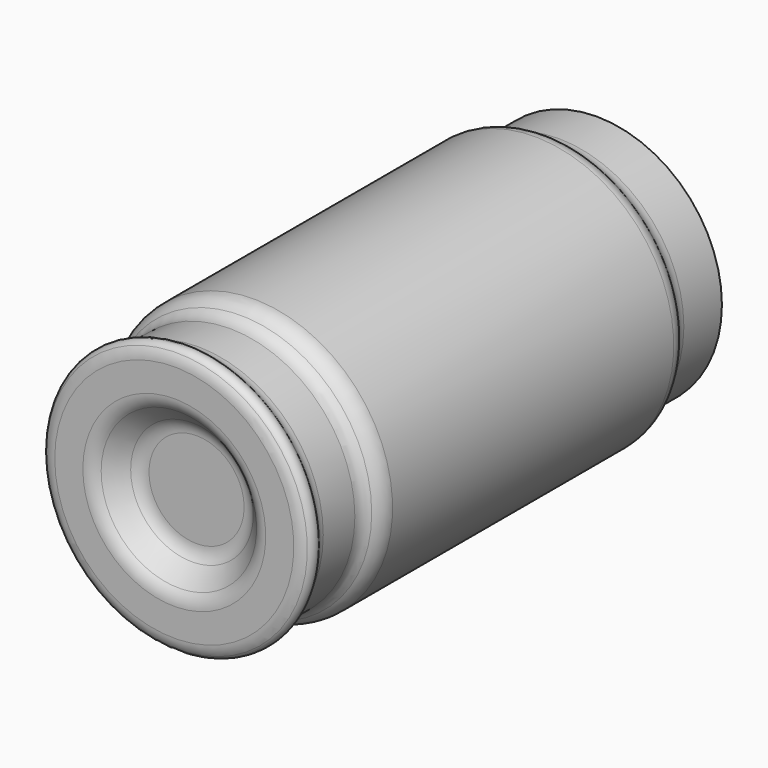
from build123d import *


# Not quite as in the source:
# - ends of sketch curves that miss each other by under 0.0002 mm in the source are joined


with BuildPart() as f1:
    # F0 (on Top) → F1 (revolve)
    with BuildSketch(Plane.XY):
        with BuildLine():
            Line((-50, 0), (-49.25, 0))
            Line((-49.25, 0), (-49.25, 67.100505))
            ThreePointArc((-49.25, 67.100505), (-48.7742470782, 69.4922764523), (-47.4194173824, 71.5199223824))
            Line((-47.4194173824, 71.5199223824), (-46.519922, 72.419417))
            ThreePointArc((-46.519922, 72.419417), (-44.839933623, 74.9336983992), (-44.25, 77.899495))
            Line((-44.25, 77.899495), (-44.25, 95))
            Line((-44.25, 95), (-45, 95))
            Line((-45, 95), (-45, 77.899495))
            ThreePointArc((-45, 77.899495), (-45.5328434077, 75.2207106468), (-47.0502530317, 72.9497470317))
            Line((-47.0502530317, 72.9497470317), (-47.949748, 72.050252))
            ThreePointArc((-47.949748, 72.050252), (-49.4671568629, 69.7792886999), (-50, 67.100505))
            Line((-50, 67.100505), (-50, 0))
        make_face()
        with BuildLine():
            Line((0, -85), (0, -84.25))
            Line((0, -84.25), (-17.100505, -84.25))
            ThreePointArc((-17.100505, -84.25), (-20.0663019275, -84.8399337583), (-22.5805830542, -86.5199229458))
            Line((-22.5805830542, -86.5199229458), (-28.480078, -92.419418))
            ThreePointArc((-28.480078, -92.419418), (-30.5077238744, -93.7742472135), (-32.899495, -94.25))
            Line((-32.899495, -94.25), (-43, -94.25))
            ThreePointArc((-43, -94.25), (-44.8261945083, -93.97724967), (-46.4929985671, -93.1828043577))
            ThreePointArc((-46.4929985671, -93.1828043577), (-47.4751196599, -91.5330711078), (-46.8265097577, -89.7260052423))
            Line((-46.8265097577, -89.7260052423), (-46.300253, -89.199748))
            ThreePointArc((-46.300253, -89.199748), (-44.7828434077, -86.9287843532), (-44.25, -84.25))
            Line((-44.25, -84.25), (-44.25, -70.04899))
            ThreePointArc((-44.25, -70.04899), (-44.9057111418, -67.090950297), (-46.7499996812, -64.6870876202))
            ThreePointArc((-46.7499996812, -64.6870876202), (-48.5942887223, -62.2832249943), (-49.25, -59.325185))
            Line((-49.25, -59.325185), (-49.25, 0))
            Line((-49.25, 0), (-50, 0))
            Line((-50, 0), (-50, -59.325185))
            ThreePointArc((-50, -59.325185), (-49.2740340482, -62.6001576243), (-47.2321430477, -65.2615770568))
            ThreePointArc((-47.2321430477, -65.2615770568), (-45.5854564677, -67.4078829271), (-45, -70.04899))
            Line((-45, -70.04899), (-45, -84.25))
            ThreePointArc((-45, -84.25), (-45.4757530571, -86.6417717789), (-46.8305831176, -88.6694178824))
            Line((-46.8305831176, -88.6694178824), (-47.35684, -89.195675))
            ThreePointArc((-47.35684, -89.195675), (-48.2216532424, -91.6050961743), (-46.9121588277, -93.8047407443))
            ThreePointArc((-46.9121588277, -93.8047407443), (-45.0453380572, -94.6945195669), (-43, -95))
            Line((-43, -95), (-32.899495, -95))
            ThreePointArc((-32.899495, -95), (-30.2207113001, -94.4671568629), (-27.9497480317, -92.9497479683))
            Line((-27.9497480317, -92.9497479683), (-22.050253, -87.050253))
            ThreePointArc((-22.050253, -87.050253), (-19.7792893532, -85.5328434077), (-17.100505, -85))
            Line((-17.100505, -85), (0, -85))
        make_face()
    revolve(axis=Axis((0, 0, 0), (0, -1, 0)))


solid = f1.part
